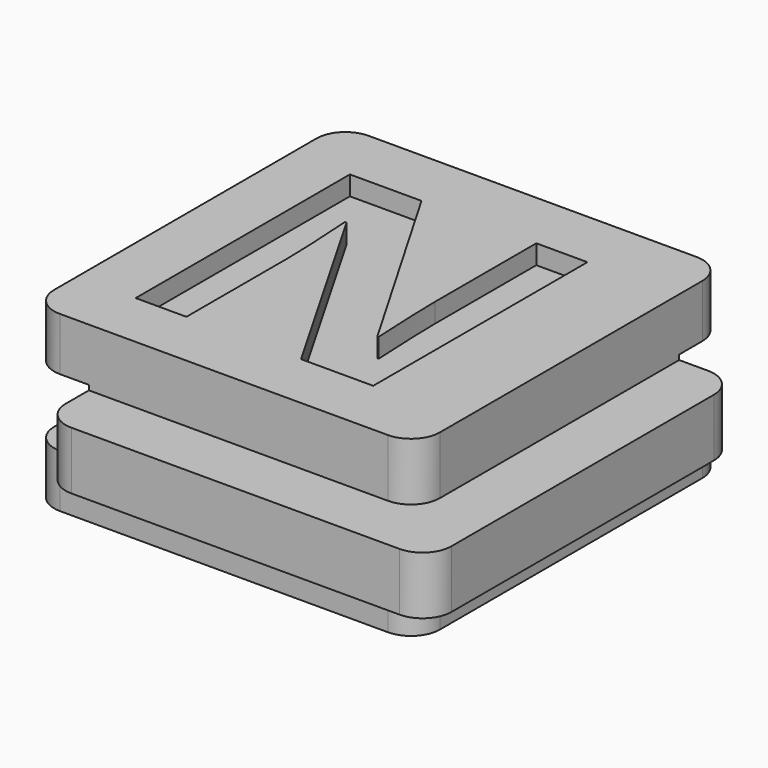
from build123d import *

# Parameters (mm, degrees)
F0_W         = 14
F0_H         = 3
F0_W_2       = 3
F1_DEPTH     = 20
F2_DEPTH     = 3
F3_W         = 3
F3_H         = 3
F4_DEPTH     = 100
F5_W         = 3
F5_H         = 3.5
F6_DEPTH     = 100
F7_R         = 1.5
F8_TEXT_SIZE = 19.4444444444
F9_DEPTH     = 1


# Not quite as in the source:
# - Text() gives the source's letters only with a copy of the font that has no kerning and outlines rounded to 1/6400 em; it was checked with that copy


with BuildPart() as f1:
    # F0 (on Front) → F1 (new body)
    with BuildSketch(Plane.XZ):
        Polygon((10, 1.5), (10, 4.5), (-10, 4.5), (-10, 1.5), (-7, 1.5), (7, 1.5), align=None)
        Rectangle(F0_W, F0_H)
        with Locations((11.5, 0)):
            Rectangle(F0_W_2, F0_H)
        with Locations((8.5, 0)):
            Rectangle(F0_W_2, F0_H)
        with Locations((-8.5, 0)):
            Rectangle(F0_W_2, F0_H)
        Polygon((10, -4.5), (10, -1.5), (7, -1.5), (-7, -1.5), (-10, -1.5), (-10, -4.5), align=None)
    extrude(amount=-F1_DEPTH)

    # F0 (on Front) → F2 (join)
    with BuildSketch(Plane.XZ):
        with Locations((-8.5, 0)):
            Rectangle(F0_W_2, F0_H)
        Rectangle(F0_W, F0_H)
        with Locations((8.5, 0)):
            Rectangle(F0_W_2, F0_H)
        with Locations((11.5, 0)):
            Rectangle(F0_W_2, F0_H)
    extrude(amount=F2_DEPTH)

    # F3 (on face) → F4 (cut)
    with BuildSketch(Plane.YZ.offset(13)):
        Polygon((23, -1.75), (23, 1.75), (17, 1.75), (17, 1.5), (20, 1.5), (20, -1.5), (17, -1.5), (17, -1.75), align=None)
        with Locations((18.5, 0)):
            Rectangle(F3_W, F3_H)
    extrude(amount=-F4_DEPTH, mode=Mode.SUBTRACT)

    # F5 (on face) → F6 (cut)
    with BuildSketch(Plane(origin=(0, 17, 0), x_dir=(-1, 0, 0), z_dir=(0, 1, 0))):
        with Locations((11.5, 0)):
            Rectangle(F5_W, F5_H)
        with Locations((8.5, 0)):
            Rectangle(F5_W, F5_H)
    extrude(amount=-F6_DEPTH, mode=Mode.SUBTRACT)

    # F7
    f7_edges = [f1.edges().sort_by_distance(p)[0] for p in [
        (-7, -3, 0),
        (13, -3, 0),
        (10, 0, 3),
        (10, 0, -3),
        (-10, 0, -3.125),
        (-10, 0, 3.125),
        (-7, 17, 0),
        (-10, 20, 3.125),
        (-10, 20, -3.125),
        (13, 17, 0),
        (10, 20, 3.125),
        (10, 20, -3.125),
    ]]
    fillet(f7_edges, radius=F7_R)

    # F8 (on face) → F9 (cut)
    with BuildSketch(Plane.XY.offset(4.5)):
        with Locations((-8.7207975495, 3)):
            Text('N', F8_TEXT_SIZE, font='Open Sans', font_style=FontStyle.BOLD, text_align=(TextAlign.LEFT, TextAlign.BOTTOM))
    extrude(amount=-F9_DEPTH, mode=Mode.SUBTRACT)


solid = f1.part
